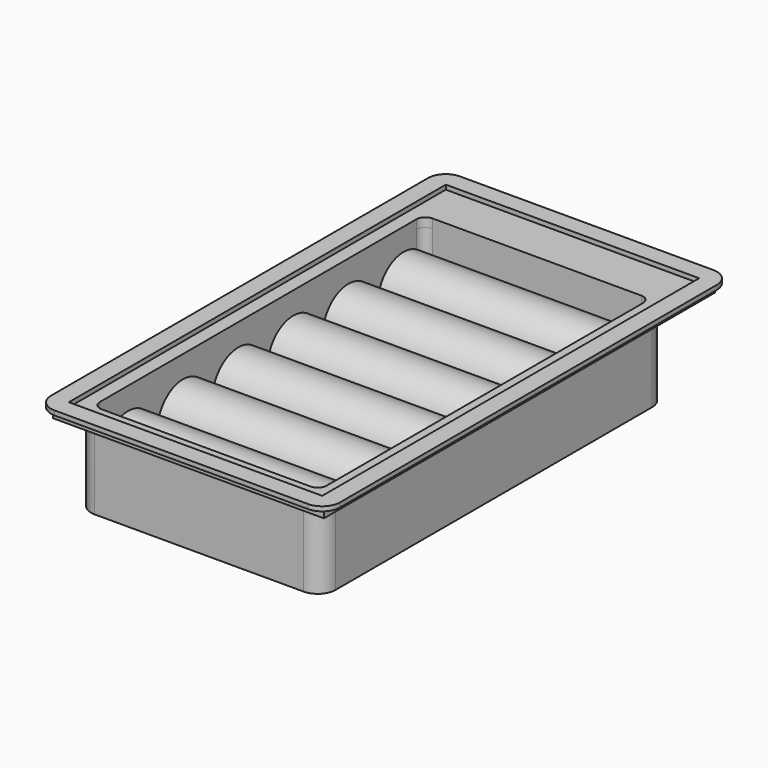
from build123d import *

# Parameters (mm, degrees)
F1_DEPTH     = 1
F2_W         = 61
F2_H         = 110
F3_DEPTH     = 2
F5_DEPTH     = 18
F6_T         = 2
F6_T3_DEPTH  = 114
F6_T5_DEPTH  = 65
F6_T7_DEPTH  = 51
F6_T9_DEPTH  = 93
F6_T12_ANGLE = 90.000000001
F6_T14_ANGLE = 90.000000001
F6_T16_ANGLE = 90.000000001
F6_T18_ANGLE = 90.000000001
F7_R         = 7.25
F8_DEPTH     = 24


# Not quite as in the source:
# - a shell that OpenCascade refuses in one call is made with other operations: the cavity is built on its own and cut out


with BuildPart() as f1:
    # F0 (on Top) → F1 (new body)
    with BuildSketch(Plane.XY):
        with BuildLine():
            ThreePointArc((32.5, 53), (31.3284271247, 55.8284271247), (28.5, 57))
            Line((28.5, 57), (-28.5, 57))
            ThreePointArc((-28.5, 57), (-31.3284271247, 55.8284271247), (-32.5, 53))
            Line((-32.5, 53), (-32.5, -53))
            ThreePointArc((-32.5, -53), (-31.3284271247, -55.8284271247), (-28.5, -57))
            Line((-28.5, -57), (28.5, -57))
            ThreePointArc((28.5, -57), (31.3284271247, -55.8284271247), (32.5, -53))
            Line((32.5, -53), (32.5, 53))
        make_face()
    extrude(amount=F1_DEPTH)

    # F2 (on Top) → F3 (join)
    with BuildSketch(Plane.XY):
        Rectangle(F2_W, F2_H)
    extrude(amount=-F3_DEPTH)

    # F4 (on face) → F5 (join)
    with BuildSketch(Plane(origin=(0, 0, -2), x_dir=(1, 0, 0), z_dir=(0, 0, -1))):
        with BuildLine():
            Line((23.5, 52), (-23.5, 52))
            ThreePointArc((-23.5, 52), (-26.3284271247, 50.8284271247), (-27.5, 48))
            Line((-27.5, 48), (-27.5, -41))
            ThreePointArc((-27.5, -41), (-26.3284271247, -43.8284271247), (-23.5, -45))
            Line((-23.5, -45), (23.5, -45))
            ThreePointArc((23.5, -45), (26.3284271247, -43.8284271247), (27.5, -41))
            Line((27.5, -41), (27.5, 48))
            ThreePointArc((27.5, 48), (26.3284271247, 50.8284271247), (23.5, 52))
        make_face()
    extrude(amount=F5_DEPTH)

    # F6: shell of thickness 2, made by hand


with BuildPart() as f6_core1:
    # F6_t2: copy of F1
    add(f1.part)

    # the walls: a layer under each face that stays
    f6_faces = [f6_core1.faces().sort_by_distance(p)[0] for p in [
        (31.3284271247, 55.8284271247, 0.5),
        (32.5, 0, 0.5),
        (0, 57, 0.5),
        (22.34375, -55.5925925926, 0),
        (31.3284271247, -55.8284271247, 0.5),
        (-31.3284271247, 55.8284271247, 0.5),
        (0, -57, 0.5),
        (-32.5, 0, 0.5),
        (-31.3284271247, -55.8284271247, 0.5),
        (30.5, 0, -1),
        (0, 55, -1),
        (-30.5, 0, -1),
        (0, -55, -1),
        (-26.1428571429, 47.1428571429, -2),
        (26.3284271247, 43.8284271247, -11),
        (0, 45, -11),
        (-26.3284271247, 43.8284271247, -11),
        (-27.5, -3.5, -11),
        (-26.3284271247, -50.8284271247, -11),
        (0, -52, -11),
        (26.3284271247, -50.8284271247, -11),
        (27.5, -3.5, -11),
        (0, -3.5, -20),
    ]]
    thicken(f6_faces, amount=-F6_T, mode=Mode.SUBTRACT)

    # F6_s4 → F6_t3 (cut)
    with BuildSketch(Plane.XZ.offset(-57)):
        Polygon((30.52, -0.02), (30.5, 2), (28.5, 2), (28.5, 0), align=None)
        Polygon((-30.52, -0.02), (-30.5, 2), (-28.5, 2), (-28.5, 0), align=None)
    extrude(amount=F6_T3_DEPTH, mode=Mode.SUBTRACT)

    # F6_s6 → F6_t5 (cut)
    with BuildSketch(Plane.YZ.offset(-32.5)):
        Polygon((55.02, -0.02), (55, 2), (53, 2), (53, 0), align=None)
        Polygon((-55.02, -0.02), (-55, 2), (-53, 2), (-53, 0), align=None)
    extrude(amount=F6_T5_DEPTH, mode=Mode.SUBTRACT)

    # F6_s8 → F6_t7 (cut)
    with BuildSketch(Plane.YZ.offset(-25.5)):
        Polygon((45.02, -2.02), (45, 0), (43, 0), (43, -2), align=None)
        Polygon((-52.02, -2.02), (-52, 0), (-50, 0), (-50, -2), align=None)
    extrude(amount=F6_T7_DEPTH, mode=Mode.SUBTRACT)

    # F6_s10 → F6_t9 (cut)
    with BuildSketch(Plane.XZ.offset(-43)):
        Polygon((-27.52, -2.02), (-27.5, 0), (-25.5, 0), (-25.5, -2), align=None)
        Polygon((27.52, -2.02), (27.5, 0), (25.5, 0), (25.5, -2), align=None)
    extrude(amount=F6_T9_DEPTH, mode=Mode.SUBTRACT)

    # F6_s11 → F6_t12 (revolve, cut)
    with BuildSketch(Plane.YZ.offset(23.5)):
        Polygon((45.02, -2.02), (45, 0), (43, 0), (43, -2), align=None)
    revolve(axis=Axis((23.5, 41, -2), (0, 0, -1)), revolution_arc=F6_T12_ANGLE, mode=Mode.SUBTRACT)

    # F6_s13 → F6_t14 (revolve, cut)
    with BuildSketch(Plane.XZ.offset(-41)):
        Polygon((-27.52, -2.02), (-27.5, 0), (-25.5, 0), (-25.5, -2), align=None)
    revolve(axis=Axis((-23.5, 41, -2), (0, 0, -1)), revolution_arc=F6_T14_ANGLE, mode=Mode.SUBTRACT)

    # F6_s15 → F6_t16 (revolve, cut)
    with BuildSketch(Plane.YZ.offset(-23.5)):
        Polygon((-52.02, -2.02), (-52, 0), (-50, 0), (-50, -2), align=None)
    revolve(axis=Axis((-23.5, -48, -2), (0, 0, -1)), revolution_arc=F6_T16_ANGLE, mode=Mode.SUBTRACT)

    # F6_s17 → F6_t18 (revolve, cut)
    with BuildSketch(Plane.XZ.offset(48)):
        Polygon((27.52, -2.02), (27.5, 0), (25.5, 0), (25.5, -2), align=None)
    revolve(axis=Axis((23.5, -48, -2), (0, 0, -1)), revolution_arc=F6_T18_ANGLE, mode=Mode.SUBTRACT)


with BuildPart() as f1_1:
    add(f1.part)

    # what is left inside the walls is the cavity
    f6_cavity = [f6_core1.part.solids().sort_by_distance(p)[0] for p in [
        (0, -17.666667, 0.98),
    ]]
    add(f6_cavity, mode=Mode.SUBTRACT)

    # F7 (on Right) → F8 (join, symmetric)
    with BuildSketch(Plane.YZ):
        with Locations((35.5, -11)):
            Circle(F7_R)
        with Locations((20, -11)):
            Circle(F7_R)
        with Locations((4.5, -11)):
            Circle(F7_R)
        with Locations((-11, -11)):
            Circle(F7_R)
        with Locations((-26.5, -11)):
            Circle(F7_R)
        with Locations((-42, -11)):
            Circle(F7_R)
    extrude(amount=F8_DEPTH, both=True)


solid = f1_1.part
